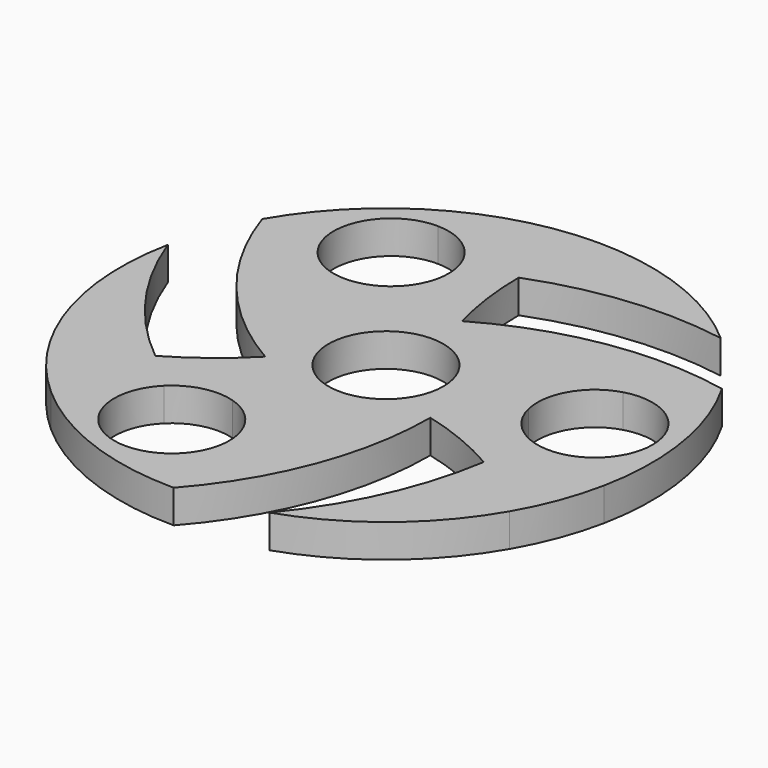
from build123d import *

# Parameters (mm, degrees)
F0_R     = 11
F1_DEPTH = 3.175
F2_DEPTH = 3.175


with BuildPart() as f1:
    # F0 (on Top) → F1 (new body, symmetric)
    with BuildSketch(Plane.XY):
        with BuildLine():
            ThreePointArc((20.292549, -3.190621), (15.603867, 0.493492), (10.5871, 3.716606))
            Line((10.5871, 3.716606), (10.5871, -14.535403))
            ThreePointArc((10.5871, -14.535403), (18.397515, -17.131664), (25.787001, -20.756393))
            ThreePointArc((25.787001, -20.756393), (32.620851, -25.343511), (38.774487, -30.809399))
            ThreePointArc((38.774487, -30.809399), (34.310981, -20.571216), (28.105483, -11.284932))
            ThreePointArc((28.105483, -11.284932), (23.085978, -8.312122), (20.292549, -3.190621))
        make_face()
        Polygon((10.5871, -14.535403), (10.5871, 3.716606), (-5.219603, 12.84261), (-21.026306, 3.716606), (-21.026306, -14.535403), (-5.219603, -23.661407), align=None)
        with Locations((-5.219603, -5.409399)):
            Circle(F0_R, mode=Mode.SUBTRACT)
        with BuildLine():
            Line((-5.219603, 12.84261), (10.5871, 3.716606))
            ThreePointArc((10.5871, 3.716606), (16.740736, 9.182493), (23.574586, 13.769612))
            ThreePointArc((23.574586, 13.769612), (30.964072, 17.39434), (38.774487, 19.990601))
            ThreePointArc((38.774487, 19.990601), (16.122412, 20.448153), (-5.219603, 12.84261))
        make_face()
        with BuildLine():
            ThreePointArc((-5.219603, -56.209399), (6.502686, -36.820901), (10.5871, -14.535403))
            Line((10.5871, -14.535403), (-5.219603, -23.661407))
            ThreePointArc((-5.219603, -23.661407), (-3.562824, -31.723556), (-3.007188, -39.935403))
            ThreePointArc((-3.007188, -39.935403), (-3.562824, -48.14725), (-5.219603, -56.209399))
        make_face()
        with BuildLine():
            Line((-21.026306, 3.716606), (-5.219603, 12.84261))
            ThreePointArc((-5.219603, 12.84261), (-6.876383, 20.904759), (-7.432019, 29.116606))
            ThreePointArc((-7.432019, 29.116606), (-6.876383, 37.328452), (-5.219603, 45.390601))
            ThreePointArc((-5.219603, 45.390601), (-11.854376, 36.406), (-16.793785, 26.388739))
            ThreePointArc((-16.793785, 26.388739), (-16.522621, 25.000927), (-16.431732, 23.589795))
            ThreePointArc((-16.431732, 23.589795), (-17.335201, 19.224012), (-19.897197, 15.575384))
            ThreePointArc((-19.897197, 15.575384), (-20.743392, 9.672811), (-21.026306, 3.716606))
        make_face()
        with BuildLine():
            ThreePointArc((38.774487, 19.990601), (30.964072, 17.39434), (23.574586, 13.769612))
            ThreePointArc((23.574586, 13.769612), (25.809021, 11.881337), (27.960245, 9.898783))
            ThreePointArc((27.960245, 9.898783), (37.61704, 8.114843), (42.0005, -0.672728))
            ThreePointArc((42.0005, -0.672728), (41.596743, -3.625628), (40.415115, -6.361755))
            ThreePointArc((40.415115, -6.361755), (42.663166, -10.833694), (44.576485, -15.458754))
            ThreePointArc((44.576485, -15.458754), (44.913356, 2.795866), (38.774487, 19.990601))
        make_face()
        with BuildLine():
            ThreePointArc((-16.054161, -28.612959), (-10.519285, -26.394499), (-5.219603, -23.661407))
            Line((-5.219603, -23.661407), (-21.026306, -14.535403))
            ThreePointArc((-21.026306, -14.535403), (-27.179942, -20.00129), (-34.013792, -24.588409))
            ThreePointArc((-34.013792, -24.588409), (-41.403278, -28.213137), (-49.213694, -30.809399))
            ThreePointArc((-49.213694, -30.809399), (-38.115414, -32.06298), (-26.970508, -31.332003))
            ThreePointArc((-26.970508, -31.332003), (-21.886226, -28.471389), (-16.054161, -28.612959))
        make_face()
        with BuildLine():
            ThreePointArc((38.774487, -30.809399), (32.620851, -25.343511), (25.787001, -20.756393))
            ThreePointArc((25.787001, -20.756393), (20.588854, -38.154406), (10.975444, -53.558754))
            ThreePointArc((10.975444, -53.558754), (26.952844, -44.723183), (38.774487, -30.809399))
        make_face()
        with BuildLine():
            ThreePointArc((-38.820645, -43.509399), (-23.180116, -52.928448), (-5.219603, -56.209399))
            ThreePointArc((-5.219603, -56.209399), (-3.562824, -48.14725), (-3.007188, -39.935403))
            ThreePointArc((-3.007188, -39.935403), (-5.759699, -40.926344), (-8.552253, -41.798082))
            ThreePointArc((-8.552253, -41.798082), (-17.801202, -50.052392), (-28.861727, -44.454046))
            ThreePointArc((-28.861727, -44.454046), (-33.858565, -44.164946), (-38.820645, -43.509399))
        make_face()
        with BuildLine():
            Line((-21.026306, -14.535403), (-21.026306, 3.716606))
            ThreePointArc((-21.026306, 3.716606), (-28.836722, 6.312867), (-36.226208, 9.937595))
            ThreePointArc((-36.226208, 9.937595), (-43.060058, 14.524714), (-49.213694, 19.990601))
            ThreePointArc((-49.213694, 19.990601), (-38.283907, 0.144553), (-21.026306, -14.535403))
        make_face()
        with BuildLine():
            ThreePointArc((-5.219603, 45.390601), (-6.876383, 37.328452), (-7.432019, 29.116606))
            ThreePointArc((-7.432019, 29.116606), (10.234176, 33.313884), (28.381438, 32.690601))
            ThreePointArc((28.381438, 32.690601), (12.740909, 42.10965), (-5.219603, 45.390601))
        make_face()
        with BuildLine():
            ThreePointArc((40.415115, -6.361755), (35.085314, -10.886165), (28.105483, -11.284932))
            ThreePointArc((28.105483, -11.284932), (34.310981, -20.571216), (38.774487, -30.809399))
            ThreePointArc((38.774487, -30.809399), (42.299445, -23.369911), (44.576485, -15.458754))
            ThreePointArc((44.576485, -15.458754), (42.663166, -10.833694), (40.415115, -6.361755))
        make_face()
        with BuildLine():
            ThreePointArc((-49.213694, -30.809399), (-44.533388, -37.581846), (-38.820645, -43.509399))
            ThreePointArc((-38.820645, -43.509399), (-33.858565, -44.164946), (-28.861727, -44.454046))
            ThreePointArc((-28.861727, -44.454046), (-30.115081, -37.576098), (-26.970508, -31.332003))
            ThreePointArc((-26.970508, -31.332003), (-38.115414, -32.06298), (-49.213694, -30.809399))
        make_face()
        with BuildLine():
            ThreePointArc((-49.213694, 19.990601), (-43.060058, 14.524714), (-36.226208, 9.937595))
            ThreePointArc((-36.226208, 9.937595), (-35.708132, 12.816811), (-35.066802, 15.671102))
            ThreePointArc((-35.066802, 15.671102), (-37.59077, 27.808082), (-27.212198, 34.587604))
            ThreePointArc((-27.212198, 34.587604), (-24.463411, 38.770444), (-21.41465, 42.739957))
            ThreePointArc((-21.41465, 42.739957), (-37.392051, 33.904386), (-49.213694, 19.990601))
        make_face()
        with BuildLine():
            ThreePointArc((-16.793785, 26.388739), (-11.854376, 36.406), (-5.219603, 45.390601))
            ThreePointArc((-5.219603, 45.390601), (-13.424868, 44.723561), (-21.41465, 42.739957))
            ThreePointArc((-21.41465, 42.739957), (-24.463411, 38.770444), (-27.212198, 34.587604))
            ThreePointArc((-27.212198, 34.587604), (-20.629043, 32.234067), (-16.793785, 26.388739))
        make_face()
        with BuildLine():
            ThreePointArc((-49.213694, -30.809399), (-41.403278, -28.213137), (-34.013792, -24.588409))
            ThreePointArc((-34.013792, -24.588409), (-46.48184, -11.387675), (-55.015692, 4.639957))
            ThreePointArc((-55.015692, 4.639957), (-55.352563, -13.614663), (-49.213694, -30.809399))
        make_face()
        with BuildLine():
            ThreePointArc((-36.226208, 9.937595), (-28.836722, 6.312867), (-21.026306, 3.716606))
            ThreePointArc((-21.026306, 3.716606), (-20.743392, 9.672811), (-19.897197, 15.575384))
            ThreePointArc((-19.897197, 15.575384), (-27.501139, 12.590014), (-35.066802, 15.671102))
            ThreePointArc((-35.066802, 15.671102), (-35.708132, 12.816811), (-36.226208, 9.937595))
        make_face()
        with BuildLine():
            ThreePointArc((23.574586, 13.769612), (16.740736, 9.182493), (10.5871, 3.716606))
            ThreePointArc((10.5871, 3.716606), (15.603867, 0.493492), (20.292549, -3.190621))
            ThreePointArc((20.292549, -3.190621), (21.509113, 4.887271), (27.960245, 9.898783))
            ThreePointArc((27.960245, 9.898783), (25.809021, 11.881337), (23.574586, 13.769612))
        make_face()
        with BuildLine():
            ThreePointArc((-3.007188, -39.935403), (-3.562824, -31.723556), (-5.219603, -23.661407))
            ThreePointArc((-5.219603, -23.661407), (-10.519285, -26.394499), (-16.054161, -28.612959))
            ThreePointArc((-16.054161, -28.612959), (-10.398433, -32.584302), (-8.227578, -39.145263))
            ThreePointArc((-8.227578, -39.145263), (-8.309048, -40.48157), (-8.552253, -41.798082))
            ThreePointArc((-8.552253, -41.798082), (-5.759699, -40.926344), (-3.007188, -39.935403))
        make_face()
    extrude(amount=F1_DEPTH, both=True)

    # F0 (on Top) → F2 (join, symmetric)
    with BuildSketch(Plane.XY):
        Polygon((10.5871, -14.535403), (10.5871, 3.716606), (-5.219603, 12.84261), (-21.026306, 3.716606), (-21.026306, -14.535403), (-5.219603, -23.661407), align=None)
        with Locations((-5.219603, -5.409399)):
            Circle(F0_R, mode=Mode.SUBTRACT)
    extrude(amount=F2_DEPTH, both=True)


solid = f1.part
